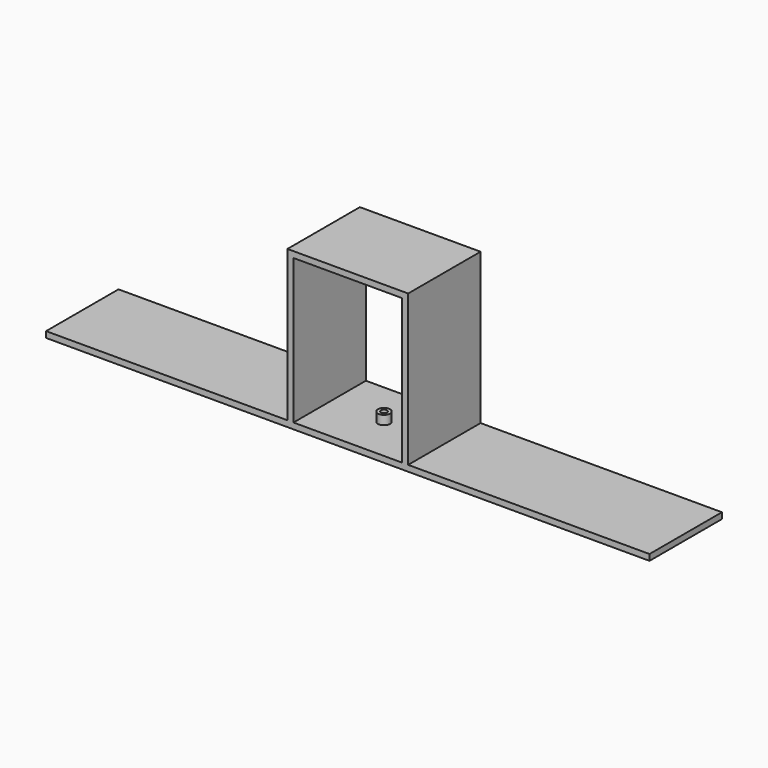
from build123d import *

# Parameters (mm, degrees)
F0_W     = 180
F0_H     = 240
F1_DEPTH = 75
F3_D     = 10
F3_DEPTH = 600
F3_TIP   = 3.0043030951
F2_R     = 10
F2_R_2   = 5
F4_DEPTH = 15


with BuildPart() as f1:
    # F0 (on Front) → F1 (new body, symmetric)
    with BuildSketch(Plane.XZ):
        Polygon((387.4092161655, 284.3629608303), (187.4092161655, 284.3629608303), (187.4092161655, 34.3629608303), (-212.5907838345, 34.3629608303), (-212.5907838345, 24.3629608303), (787.4092161655, 24.3629608303), (787.4092161655, 34.3629608303), (387.4092161655, 34.3629608303), align=None)
        with Locations((287.4092161655, 154.3629608303)):
            Rectangle(F0_W, F0_H, mode=Mode.SUBTRACT)
    extrude(amount=F1_DEPTH, both=True)

    # F3 (one way)
    with BuildSketch(Plane.XY.offset(34.3629608303)):
        with Locations((287.4092161655, 0)):
            Circle(F3_D / 2)
    extrude(amount=-F3_DEPTH, mode=Mode.SUBTRACT)
    with Locations(Plane.XY.offset(34.3629608303)):
        with Locations((287.4092161655, 0)):
            with Locations((0, 0, -(F3_DEPTH + F3_TIP / 2))):  # 118° drill point
                Cone(0, F3_D / 2, F3_TIP, mode=Mode.SUBTRACT)

    # F2 (on face) → F4 (join)
    with BuildSketch(Plane.XY.offset(34.3629608303)):
        with Locations((287.4092161655, 0)):
            Circle(F2_R)
        with Locations((287.4092161655, 0)):
            Circle(F2_R_2, mode=Mode.SUBTRACT)
    extrude(amount=F4_DEPTH)


solid = f1.part
